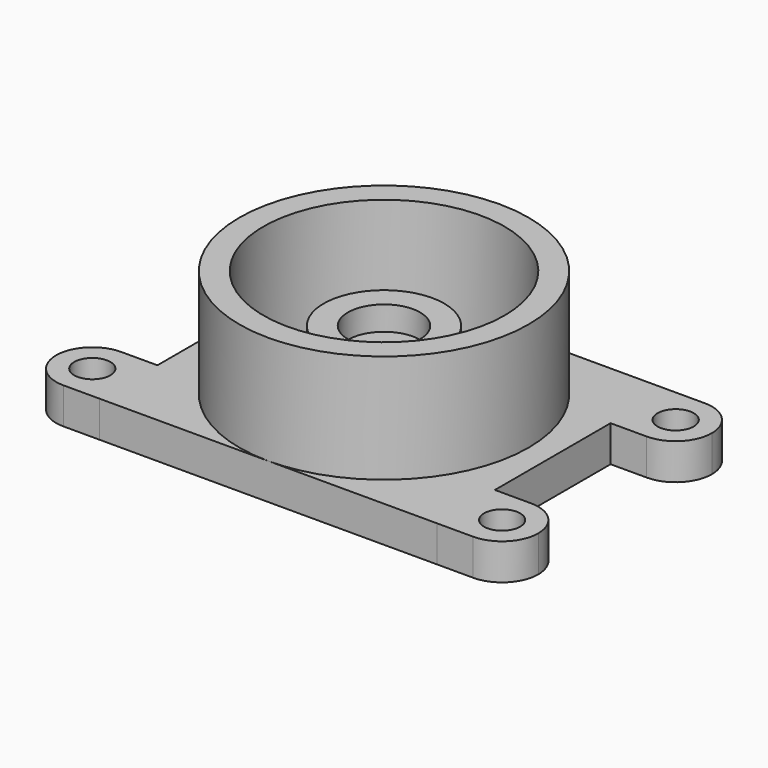
from build123d import *

# Parameters (mm, degrees)
F0_R     = 63.5
F0_R_2   = 9.525
F0_R_3   = 31.75
F0_R_4   = 19.05
F1_DEPTH = 19.05
F2_DEPTH = 57.15
F3_DEPTH = 31.75
F4_DEPTH = 19.05
F5_DEPTH = 25.4


# Not quite as in the source:
# - ends of sketch curves that miss each other by under 0.0002 mm in the source are joined


with BuildPart() as f1:
    # F0 (on Top) → F1 (new body)
    with BuildSketch(Plane.XY):
        with BuildLine():
            ThreePointArc((2.2517e-06, -76.2), (53.8815375225, -53.8815359303), (76.2, 0))
            ThreePointArc((76.2, 0), (53.8815360903, 53.8815373625), (-1.7992e-06, 76.2))
            ThreePointArc((-1.7992e-06, 76.2), (-76.2, -2.0255e-06), (2.2517e-06, -76.2))
        make_face()
        Circle(F0_R, mode=Mode.SUBTRACT)
        with BuildLine():
            ThreePointArc((-1.7992e-06, 76.2), (53.8815360903, 53.8815373625), (76.2, 0))
            ThreePointArc((76.2, 0), (53.8815375225, -53.8815359303), (2.2517e-06, -76.2))
            Line((2.2517e-06, -76.2), (88.9, -76.199992084))
            Line((88.9, -76.199992084), (88.9, -38.100007916))
            Line((88.9, -38.100007916), (88.9, 38.100007916))
            Line((88.9, 38.100007916), (88.9, 76.200007916))
            Line((88.9, 76.200007916), (-1.7992e-06, 76.2))
        make_face()
        with BuildLine():
            ThreePointArc((2.2517e-06, -76.2), (-76.2, -2.0255e-06), (-1.7992e-06, 76.2))
            Line((-1.7992e-06, 76.2), (-88.9, 76.199992084))
            Line((-88.9, 76.199992084), (-88.9, 38.100007916))
            Line((-88.9, 38.100007916), (-88.9, -38.100007916))
            Line((-88.9, -38.100007916), (-88.9, -76.200007916))
            Line((-88.9, -76.200007916), (2.2517e-06, -76.2))
        make_face()
        with BuildLine():
            Line((-88.9, 38.100007916), (-88.9, 76.199992084))
            Line((-88.9, 76.199992084), (-107.95, 76.200007916))
            ThreePointArc((-107.95, 76.200007916), (-121.4203841816, 70.6203920976), (-127, 57.150007916))
            ThreePointArc((-127, 57.150007916), (-121.4203841816, 43.6796237344), (-107.95, 38.100007916))
            Line((-107.95, 38.100007916), (-88.9, 38.100007916))
        make_face()
        with Locations((-107.95, 57.150007916)):
            Circle(F0_R_2, mode=Mode.SUBTRACT)
        with BuildLine():
            Line((107.95, 76.200007916), (88.9, 76.200007916))
            Line((88.9, 76.200007916), (88.9, 38.100007916))
            Line((88.9, 38.100007916), (107.95, 38.100007916))
            ThreePointArc((107.95, 38.100007916), (121.4203841816, 43.6796237344), (127, 57.150007916))
            ThreePointArc((127, 57.150007916), (121.4203841816, 70.6203920976), (107.95, 76.200007916))
        make_face()
        with Locations((107.95, 57.150007916)):
            Circle(F0_R_2, mode=Mode.SUBTRACT)
        with BuildLine():
            Line((88.9, -38.100007916), (88.9, -76.199992084))
            Line((88.9, -76.199992084), (107.95, -76.200007916))
            ThreePointArc((107.95, -76.200007916), (121.4203841816, -70.6203920976), (127, -57.150007916))
            ThreePointArc((127, -57.150007916), (121.4203841816, -43.6796237344), (107.95, -38.100007916))
            Line((107.95, -38.100007916), (88.9, -38.100007916))
        make_face()
        with Locations((107.95, -57.150007916)):
            Circle(F0_R_2, mode=Mode.SUBTRACT)
        with BuildLine():
            Line((-107.95, -76.200007916), (-88.9, -76.200007916))
            Line((-88.9, -76.200007916), (-88.9, -38.100007916))
            Line((-88.9, -38.100007916), (-107.95, -38.100007916))
            ThreePointArc((-107.95, -38.100007916), (-121.4203841816, -43.6796237344), (-127, -57.150007916))
            ThreePointArc((-127, -57.150007916), (-121.4203841816, -70.6203920976), (-107.95, -76.200007916))
        make_face()
        with Locations((-107.95, -57.150007916)):
            Circle(F0_R_2, mode=Mode.SUBTRACT)
        Circle(F0_R)
        Circle(F0_R_3, mode=Mode.SUBTRACT)
        Circle(F0_R_3)
        Circle(F0_R_4, mode=Mode.SUBTRACT)
        Circle(F0_R_4)
        Circle(F0_R_2, mode=Mode.SUBTRACT)
        Circle(F0_R_2)
    extrude(amount=-F1_DEPTH)

    # F0 (on Top) → F2 (join)
    with BuildSketch(Plane.XY):
        with BuildLine():
            ThreePointArc((2.2517e-06, -76.2), (53.8815375225, -53.8815359303), (76.2, 0))
            ThreePointArc((76.2, 0), (53.8815360903, 53.8815373625), (-1.7992e-06, 76.2))
            ThreePointArc((-1.7992e-06, 76.2), (-76.2, -2.0255e-06), (2.2517e-06, -76.2))
        make_face()
        Circle(F0_R, mode=Mode.SUBTRACT)
    extrude(amount=F2_DEPTH)

    # F0 (on Top) → F3 (join)
    with BuildSketch(Plane.XY):
        Circle(F0_R_3)
        Circle(F0_R_4, mode=Mode.SUBTRACT)
    extrude(amount=F3_DEPTH)

    # F0 (on Top) → F4 (join)
    with BuildSketch(Plane.XY):
        Circle(F0_R_4)
        Circle(F0_R_2, mode=Mode.SUBTRACT)
    extrude(amount=F4_DEPTH)

    # F0 (on Top) → F5 (cut)
    with BuildSketch(Plane.XY):
        Circle(F0_R_2)
    extrude(amount=-F5_DEPTH, mode=Mode.SUBTRACT)


solid = f1.part
